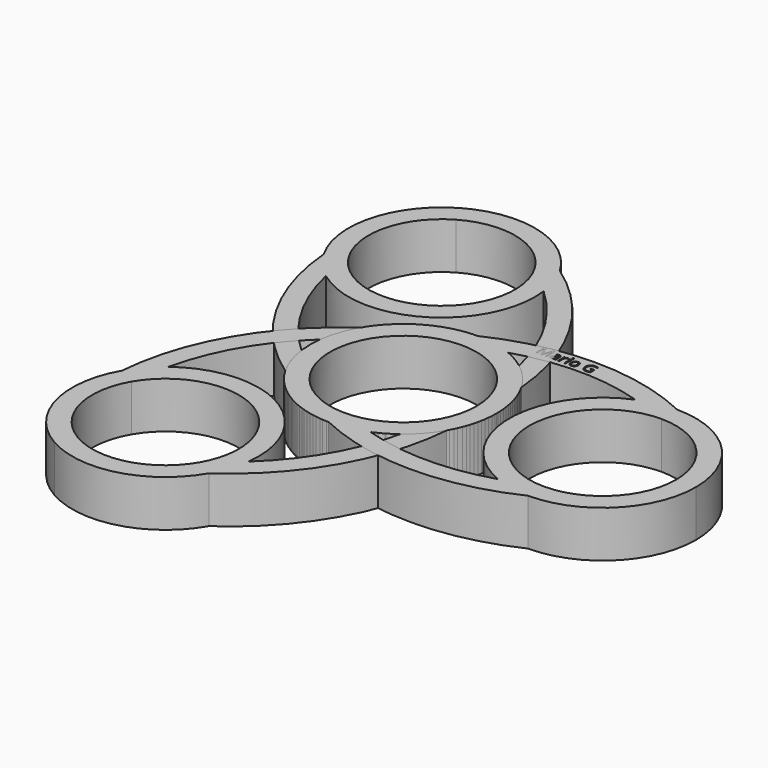
from build123d import *

# Parameters (mm, degrees)
F0_R         = 11.025
F1_DEPTH     = 7
F2_COUNT     = 3
F3_TEXT_SIZE = 2.2989297589
F4_DEPTH     = 20


# Not quite as in the source:
# - Text() gives the source's letters only with a copy of the font that has no kerning and outlines rounded to 1/6400 em; it was checked with that copy


with BuildPart() as f1:
    # F0 (on Top) → F1 (new body)
    with BuildSketch(Plane.XY):
        with BuildLine():
            ThreePointArc((44.025, 0), (39.9171726061, 9.9171726061), (30, 14.025))
            Line((30, 14.025), (30, 11.025))
            ThreePointArc((30, 11.025), (37.7958522626, 7.7958522626), (41.025, 0))
            ThreePointArc((41.025, 0), (37.7958522626, -7.7958522626), (30, -11.025))
            Line((30, -11.025), (30, -14.025))
            ThreePointArc((30, -14.025), (39.9171726061, -9.9171726061), (44.025, 0))
        make_face()
        with BuildLine():
            Line((30, 11.025), (30, 14.025))
            ThreePointArc((30, 14.025), (27.2351803861, 13.7497780892), (24.5788725636, 12.9349140824))
            ThreePointArc((24.5788725636, 12.9349140824), (15.975, 0), (24.5788725636, -12.9349140824))
            ThreePointArc((24.5788725636, -12.9349140824), (27.2351803861, -13.7497780892), (30, -14.025))
            Line((30, -14.025), (30, -11.025))
            ThreePointArc((30, -11.025), (18.975, 0), (30, 11.025))
        make_face()
        with BuildLine():
            ThreePointArc((30, 14.025), (15, 17.4022233983), (0, 14.025))
            ThreePointArc((0, 14.025), (2.7648196139, 13.7497780892), (5.4211274364, 12.9349140824))
            ThreePointArc((5.4211274364, 12.9349140824), (15, 14.4022233983), (24.5788725636, 12.9349140824))
            ThreePointArc((24.5788725636, 12.9349140824), (27.2351803861, 13.7497780892), (30, 14.025))
        make_face()
        with BuildLine():
            ThreePointArc((5.4211274364, -12.9349140824), (2.7648196139, -13.7497780892), (0, -14.025))
            ThreePointArc((0, -14.025), (15, -17.4022233983), (30, -14.025))
            ThreePointArc((30, -14.025), (27.2351803861, -13.7497780892), (24.5788725636, -12.9349140824))
            ThreePointArc((24.5788725636, -12.9349140824), (15, -14.4022233983), (5.4211274364, -12.9349140824))
        make_face()
        with BuildLine():
            ThreePointArc((5.4211274364, 12.9349140824), (2.7648196139, 13.7497780892), (0, 14.025))
            ThreePointArc((0, 14.025), (-14.025, 0), (0, -14.025))
            ThreePointArc((0, -14.025), (2.7648196139, -13.7497780892), (5.4211274364, -12.9349140824))
            ThreePointArc((5.4211274364, -12.9349140824), (11.6775840244, -7.767538629), (14.025, 0))
            ThreePointArc((14.025, 0), (11.6775840244, 7.767538629), (5.4211274364, 12.9349140824))
        make_face()
        Circle(F0_R, mode=Mode.SUBTRACT)
    extrude(amount=F1_DEPTH)


with BuildPart() as f2_1:
    # F2: instance of F1
    add(f1.part.rotate(Axis((0, 0, 7), (0, 0, 1)), 1 * 360 / F2_COUNT))


with BuildPart() as f2_2:
    # F2: instance of F1
    add(f1.part.rotate(Axis((0, 0, 7), (0, 0, 1)), 2 * 360 / F2_COUNT))


with BuildPart() as f1_1:
    add(f1.part)

    # F3 (on face) → F4 (cut)
    with BuildSketch(Plane.XY.offset(7)):
        with Locations((7.733869823, 14.9844493717)):
            Text('Mario G', F3_TEXT_SIZE, font='Open Sans', text_align=(TextAlign.LEFT, TextAlign.BOTTOM))
    extrude(amount=-F4_DEPTH, mode=Mode.SUBTRACT)


solid = Compound([f2_1.part, f2_2.part, f1_1.part])
